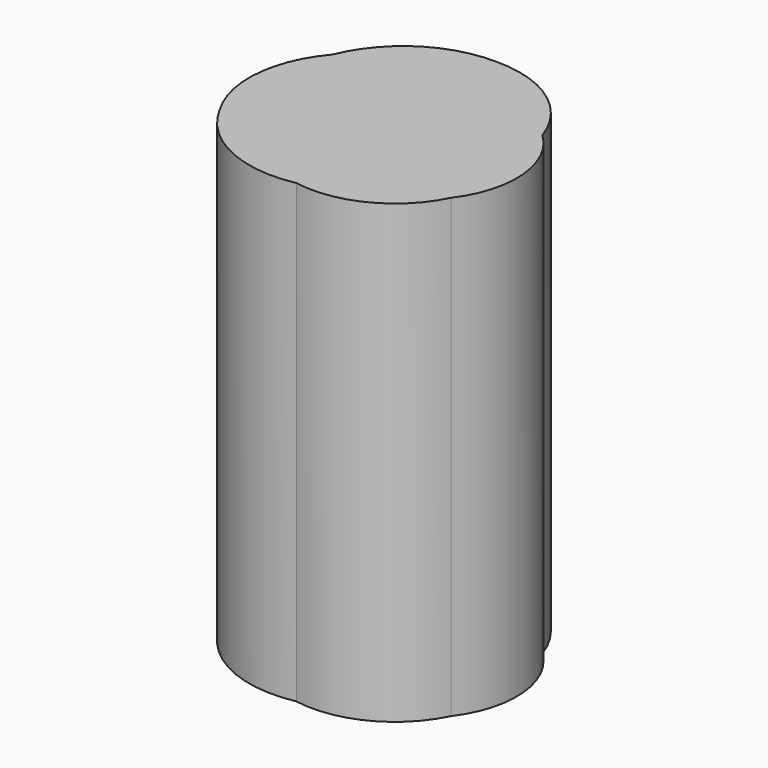
from build123d import *

# Parameters (mm, degrees)
F1_DEPTH = 7.9375


# Not quite as in the source:
# - a length typed as a fraction of an inch, garbled in the dataset ("3 / 203.2 mm" for 3/8 in), is restored


with BuildPart() as f1:
    # F0 (on Top) → F1 (new body)
    with BuildSketch(Plane.XY):
        with BuildLine():
            ThreePointArc((1.7291457625, 1.0868449463), (1.025201219, 2.031415161), (-0.1001062337, 2.3798889015))
            ThreePointArc((-0.1001062337, 2.3798889015), (-1.2304943591, 2.0620113015), (-1.9774150234, 1.155957769))
            ThreePointArc((-1.9774150234, 1.155957769), (-2.4307372074, 0.0714217097), (-2.1580981556, -1.0719887214))
            ThreePointArc((-2.1580981556, -1.0719887214), (-1.2501182209, -1.9455907072), (0, -2.1031103097))
            ThreePointArc((0, -2.1031103097), (1.1187867589, -1.9348458875), (1.9124085084, -1.1285201181))
            ThreePointArc((1.9124085084, -1.1285201181), (2.2442264135, 0.0141916193), (1.7291457625, 1.0868449463))
        make_face()
    extrude(amount=F1_DEPTH)


solid = f1.part
